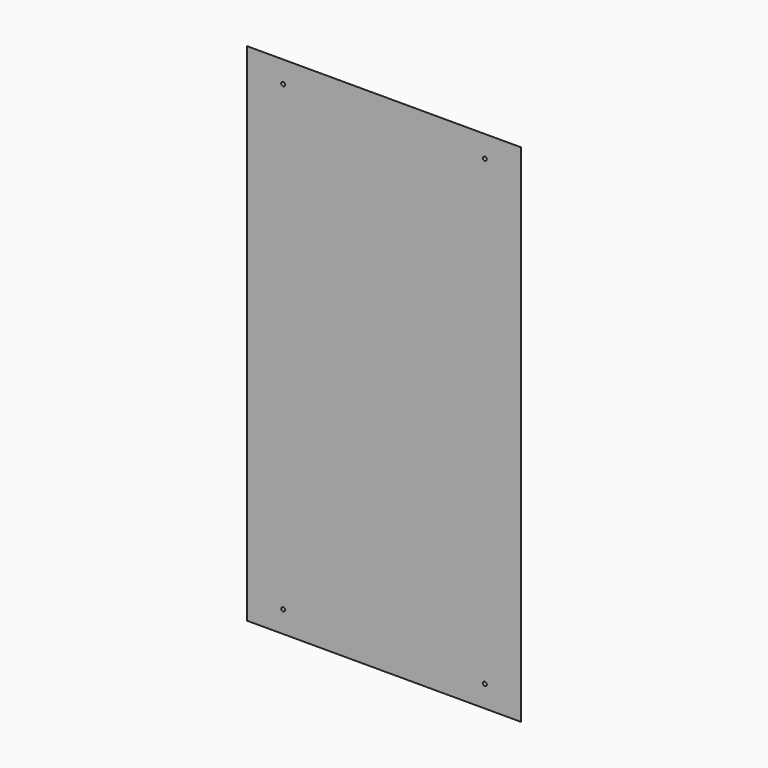
from build123d import *

# Parameters (mm, degrees)
F0_W     = 246
F0_H     = 454
F1_DEPTH = 12
F2_SIZE  = 11.99999
F4_D     = 3.5


# Not quite as in the source:
# - a fillet or chamfer is up to 0.001 mm smaller than in the source, because OpenCascade refuses the exact size


with BuildPart() as f1:
    # F0 (on Front) → F1 (new body)
    with BuildSketch(Plane.XZ):
        Rectangle(F0_W, F0_H)
    extrude(amount=F1_DEPTH)

    # F2 (size 12 in the source; OpenCascade refuses exactly that, so slightly less here)
    f2_edges = [f1.edges().sort_by_distance(p)[0] for p in [
        (0, 0, 227),
        (-123, 0, 0),
        (0, 0, -227),
        (123, 0, 0),
    ]]
    chamfer(f2_edges, length=F2_SIZE)

    # F4 (through all)
    with Locations(Plane.XZ.offset(12)):
        with Locations((-90.5, 207.5), (90.5, 207.5), (90.5, -207.5), (-90.5, -207.5)):
            Hole(F4_D / 2)


solid = f1.part
